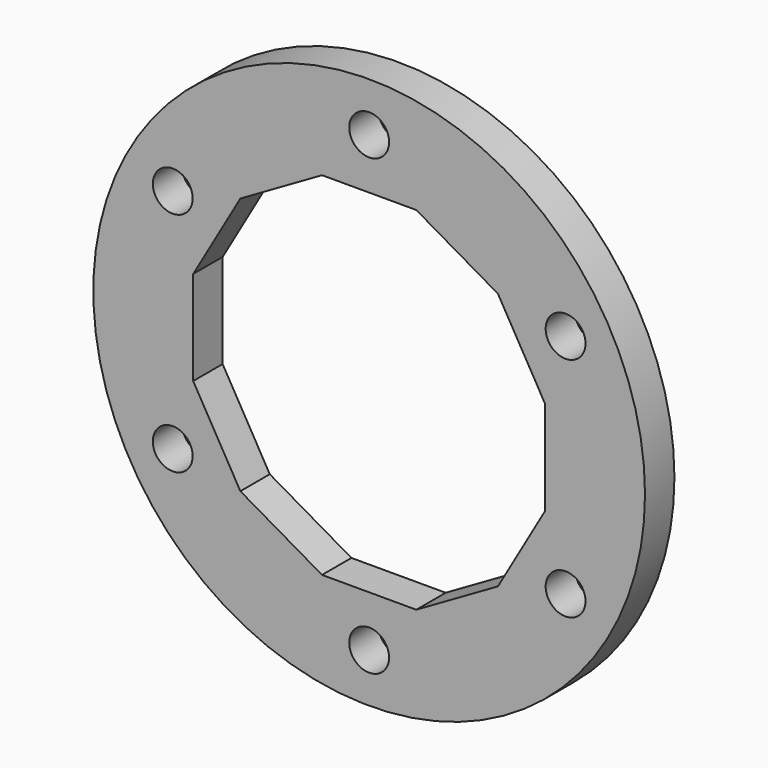
from build123d import *

# Parameters (mm, degrees)
F0_R            = 45
F1_DEPTH        = 6
F2_R            = 3.25
F3_DEPTH        = 12.5
F3_COPIES_COUNT = 6


# Not quite as in the source:
# - a pattern or mirror of a feature is missing from the dataset's text; its kind, count and spacing are read off the source's solid


with BuildPart() as f1:
    # F0 (on Front) → F1 (new body)
    with BuildSketch(Plane.XZ):
        Circle(F0_R)
        Polygon((-21.0098581772, 21.0098581772), (-7.6901418228, 28.7), (7.6901418228, 28.7), (21.0098581772, 21.0098581772), (28.7, 7.6901418228), (28.7, -7.6901418228), (21.0098581772, -21.0098581772), (7.6901418228, -28.7), (-7.6901418228, -28.7), (-21.0098581772, -21.0098581772), (-28.7, -7.6901418228), (-28.7, 7.6901418228), align=None, mode=Mode.SUBTRACT)
    extrude(amount=F1_DEPTH)

    # F2 (on face) → F3 (cut, symmetric)
    with BuildSketch(Plane.XZ.offset(6)):
        with Locations((0, 37)):
            Circle(F2_R)
    f3 = extrude(amount=F3_DEPTH, both=True, mode=Mode.SUBTRACT)

    # F3_copies: F3 ×6 about axis
    f3_copies_axis = Axis((0, 0, 0), (0, 1, 0))
    for i in range(1, F3_COPIES_COUNT):
        add(f3.rotate(f3_copies_axis, i * 360 / F3_COPIES_COUNT), mode=Mode.SUBTRACT)


solid = f1.part
